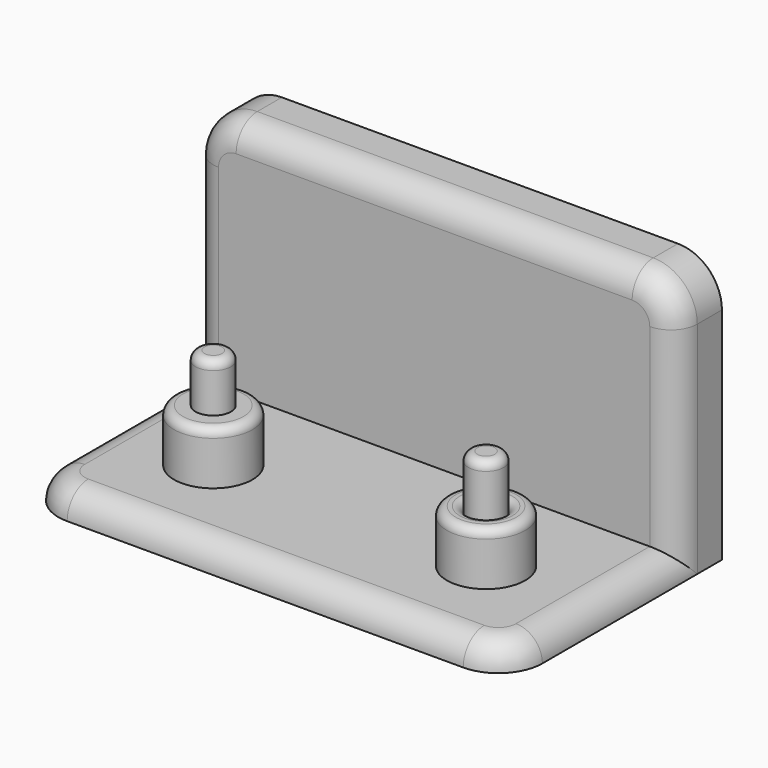
from build123d import *

# Parameters (mm, degrees)
F0_R     = 2
F1_DEPTH = 14.5
F0_R_2   = 4.45
F2_DEPTH = 9
F0_W     = 55
F0_H     = 24
F3_DEPTH = 3
F4_W     = 55
F4_H     = 27
F4_H_2   = 3
F5_DEPTH = 2
F7_DEPTH = 2.5
F9_DEPTH = 2
F10_R    = 5
F11_R    = 2.99999
F12_R    = 1
F12_2_R  = 1
F12_3_R  = 1
F12_4_R  = 1
F13_SIZE = 2


# Not quite as in the source:
# - a fillet or chamfer is up to 0.001 mm smaller than in the source, because OpenCascade refuses the exact size


with BuildPart() as f1:
    # F0 (on Top) → F1 (new body)
    with BuildSketch(Plane.XY):
        with Locations((-15.5, 0)):
            Circle(F0_R)
    extrude(amount=F1_DEPTH)

    # F12
    f12_edges = [f1.edges().sort_by_distance(p)[0] for p in [
        (-17.5, 0, 14.5),
    ]]
    fillet(f12_edges, radius=F12_R)


with BuildPart() as f1b:
    # F0 (on Top) → F1, piece 2 (new body)
    with BuildSketch(Plane.XY):
        with Locations((15.5, 0)):
            Circle(F0_R)
    extrude(amount=F1_DEPTH)

    # F12#3
    f12_3_edges = [f1b.edges().sort_by_distance(p)[0] for p in [
        (13.5, 0, 14.5),
    ]]
    fillet(f12_3_edges, radius=F12_3_R)


with BuildPart() as f2:
    # F0 (on Top) → F2 (new body)
    with BuildSketch(Plane.XY):
        with Locations((15.5, 0)):
            Circle(F0_R_2)
        with Locations((15.5, 0)):
            Circle(F0_R, mode=Mode.SUBTRACT)
    extrude(amount=F2_DEPTH)

    # F12#4
    f12_4_edges = [f2.edges().sort_by_distance(p)[0] for p in [
        (11.05, 0, 9),
        (13.5, 0, 9),
    ]]
    fillet(f12_4_edges, radius=F12_4_R)


with BuildPart() as f2b:
    # F0 (on Top) → F2, piece 2 (new body)
    with BuildSketch(Plane.XY):
        with Locations((-15.5, 0)):
            Circle(F0_R_2)
        with Locations((-15.5, 0)):
            Circle(F0_R, mode=Mode.SUBTRACT)
    extrude(amount=F2_DEPTH)

    # F12#2
    f12_2_edges = [f2b.edges().sort_by_distance(p)[0] for p in [
        (-19.95, 0, 9),
    ]]
    fillet(f12_2_edges, radius=F12_2_R)


with BuildPart() as f3:
    # F0 (on Top) → F3 (new body)
    with BuildSketch(Plane.XY):
        Rectangle(F0_W, F0_H)
        with Locations((-15.5, 0)):
            Circle(F0_R_2, mode=Mode.SUBTRACT)
        with Locations((15.5, 0)):
            Circle(F0_R_2, mode=Mode.SUBTRACT)
    extrude(amount=F3_DEPTH)

    # F4 (on face) → F5 (join)
    with BuildSketch(Plane(origin=(0, 12, 0), x_dir=(-1, 0, 0), z_dir=(0, 1, 0))):
        with Locations((0, 16.5)):
            Rectangle(F4_W, F4_H)
        with Locations((0, 1.5)):
            Rectangle(F4_W, F4_H_2)
    extrude(amount=F5_DEPTH)

    # F6 (on face) → F7 (join)
    with BuildSketch(Plane(origin=(0, 14, 0), x_dir=(-1, 0, 0), z_dir=(0, 1, 0))):
        Polygon((-27.5, 30), (-27.5, 0), (-25, 0), (-25, 27.5), (25, 27.5), (25, 0), (27.5, 0), (27.5, 30), align=None)
    extrude(amount=F7_DEPTH)

    # F8 (on face) → F9 (join)
    with BuildSketch(Plane(origin=(0, 16.5, 0), x_dir=(-1, 0, 0), z_dir=(0, 1, 0))):
        Polygon((-25, 27.5), (-25, 0), (-21.5, 0), (-21.5, 24), (21.5, 24), (21.5, 0), (25, 0), (25, 27.5), align=None)
        Polygon((-27.5, 30), (-27.5, 0), (-25, 0), (-25, 27.5), (25, 27.5), (25, 0), (27.5, 0), (27.5, 30), align=None)
    extrude(amount=F9_DEPTH)

    # F10
    f10_edges = [f3.edges().sort_by_distance(p)[0] for p in [
        (27.5, 15.25, 30),
        (-27.5, 15.25, 30),
        (-27.5, -12, 1.5),
        (27.5, -12, 1.5),
    ]]
    fillet(f10_edges, radius=F10_R)

    # F11 (radius 3 in the source; OpenCascade refuses exactly that, so slightly less here)
    f11_edges = [f3.edges().sort_by_distance(p)[0] for p in [
        (0, -12, 3),
        (0, 12, 30),
    ]]
    fillet(f11_edges, radius=F11_R)

    # F13
    f13_edges = [f3.edges().sort_by_distance(p)[0] for p in [
        (-21.5, 17.5, 0),
        (21.5, 17.5, 0),
    ]]
    chamfer(f13_edges, length=F13_SIZE)


solid = Compound([f1.part, f1b.part, f2.part, f2b.part, f3.part])
